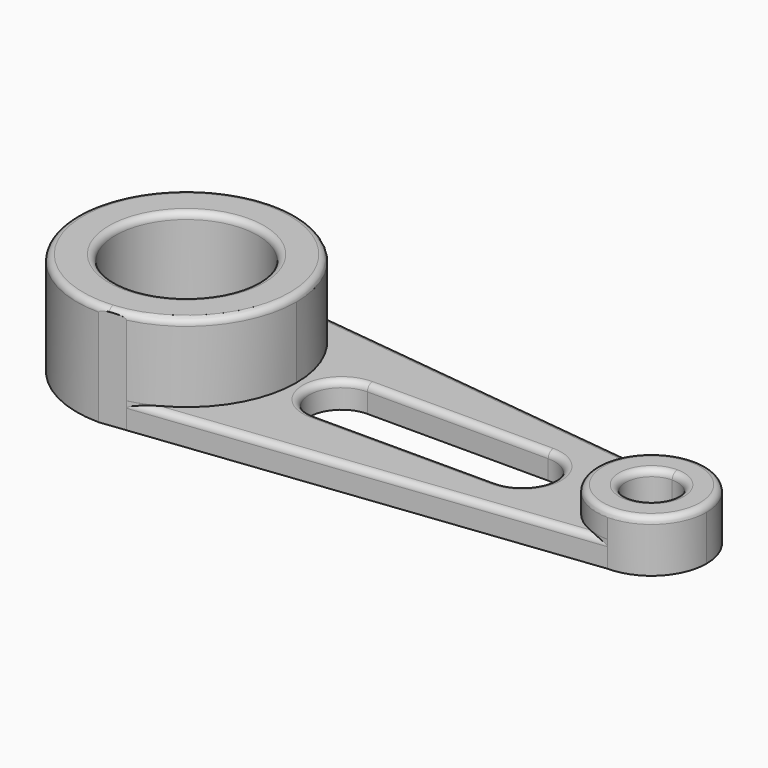
from build123d import *

# Parameters (mm, degrees)
F0_R         = 34.925
F1_DEPTH     = 50.8
F2_DEPTH     = 12.7
F3_DEPTH     = 25.4
F4_T2_ANGLE  = 170.0024112312
F4_T4_ANGLE  = 196.8788005765
F4_T8_DEPTH  = 281.0532283158
F4_S9_R      = 27.051
F4_T10_DEPTH = 142
F4_S11_R     = 53.975
F4_T12_DEPTH = 142
F4_T16_DEPTH = 281.0532283158
F4_S17_R     = 27.051
F4_T18_DEPTH = 142
F4_S19_R     = 53.975
F4_T20_DEPTH = 142
F5_R         = 3.175


# Not quite as in the source:
# - a fillet or chamfer that OpenCascade refuses, or shapes differently, is made with other operations: its cross-section is extruded or revolved along the edge and cut away or added


with BuildPart() as f1:
    # F0 (on Top) → F1 (new body)
    with BuildSketch(Plane.XY):
        with BuildLine():
            Line((-131.9052666893, 52.4980479424), (-144.4454256691, 53.975))
            ThreePointArc((-144.4454256691, 53.975), (-198.4204256691, 0), (-144.4454256691, -53.975))
            Line((-144.4454256691, -53.975), (-131.9052666893, -52.4980479424))
            ThreePointArc((-131.9052666893, -52.4980479424), (-102.0770665674, -33.4398380981), (-90.4704256691, 0))
            ThreePointArc((-90.4704256691, 0), (-102.0770665674, 33.4398380981), (-131.9052666893, 52.4980479424))
        make_face()
        with Locations((-144.4454256691, 0)):
            Circle(F0_R, mode=Mode.SUBTRACT)
    extrude(amount=F1_DEPTH)

    # F0 (on Top) → F2 (join)
    with BuildSketch(Plane.XY):
        with BuildLine():
            Line((84.1545743309, 27.051), (-131.9052666893, 52.4980479424))
            ThreePointArc((-131.9052666893, 52.4980479424), (-102.0770665674, 33.4398380981), (-90.4704256691, 0))
            ThreePointArc((-90.4704256691, 0), (-102.0770665674, -33.4398380981), (-131.9052666893, -52.4980479424))
            Line((-131.9052666893, -52.4980479424), (84.1545743309, -27.051))
            ThreePointArc((84.1545743309, -27.051), (57.1035743309, 0), (84.1545743309, 27.051))
        make_face()
        with BuildLine():
            ThreePointArc((-68.2454256691, -15.875), (-84.1204256691, 0), (-68.2454256691, 15.875))
            Line((-68.2454256691, 15.875), (20.6545743309, 15.875))
            ThreePointArc((20.6545743309, 15.875), (36.5295743309, 0), (20.6545743309, -15.875))
            Line((20.6545743309, -15.875), (-68.2454256691, -15.875))
        make_face(mode=Mode.SUBTRACT)
    extrude(amount=F2_DEPTH)

    # F0 (on Top) → F3 (join)
    with BuildSketch(Plane.XY):
        with BuildLine():
            ThreePointArc((111.2055743309, 0), (103.2825198687, 19.1279455379), (84.1545743309, 27.051))
            Line((84.1545743309, 27.051), (84.1545743309, 12.7))
            ThreePointArc((84.1545743309, 12.7), (93.1348304519, 8.9802561211), (96.8545743309, 0))
            ThreePointArc((96.8545743309, 0), (93.1348304519, -8.9802561211), (84.1545743309, -12.7))
            Line((84.1545743309, -12.7), (84.1545743309, -27.051))
            ThreePointArc((84.1545743309, -27.051), (103.2825198687, -19.1279455379), (111.2055743309, 0))
        make_face()
        with BuildLine():
            Line((84.1545743309, 12.7), (84.1545743309, 27.051))
            ThreePointArc((84.1545743309, 27.051), (57.1035743309, 0), (84.1545743309, -27.051))
            Line((84.1545743309, -27.051), (84.1545743309, -12.7))
            ThreePointArc((84.1545743309, -12.7), (71.4545743309, 0), (84.1545743309, 12.7))
        make_face()
    extrude(amount=F3_DEPTH)

    # F4: fillet of radius 3.175 on 5 edges, made by hand

    # F4_s1 → F4_t2 (revolve, cut)
    with BuildSketch(Plane(origin=(-143.3487281035, 12.5383492192, 0), x_dir=(0, 0, 1), z_dir=(-0.9961965318, 0.0871347808, 0))):
        with BuildLine():
            ThreePointArc((47.625, 41.3887794913), (49.8700640303, 40.4588435216), (50.8, 38.2137794913))
            Line((50.8, 38.2137794913), (50.8635, 38.2137794913))
            Line((50.8635, 38.2137794913), (50.8635, 41.4522794913))
            Line((50.8635, 41.4522794913), (47.625, 41.4522794913))
            Line((47.625, 41.4522794913), (47.625, 41.3887794913))
        make_face()
    revolve(axis=Axis((-144.4454256691, 0, 50.8), (0, 0, -1)), revolution_arc=F4_T2_ANGLE, mode=Mode.SUBTRACT)

    # F4_s3 → F4_t4 (revolve, cut)
    with BuildSketch(Plane(origin=(-141.3341490778, 20.9697312712, 0), x_dir=(0, 0, 1), z_dir=(0.9891716429, -0.1467632817, 0))):
        with BuildLine():
            ThreePointArc((50.8, -29.6007153042), (49.8700640303, -31.8457793344), (47.625, -32.7757153042))
            Line((47.625, -32.7757153042), (47.625, -32.8392153042))
            Line((47.625, -32.8392153042), (50.8635, -32.8392153042))
            Line((50.8635, -32.8392153042), (50.8635, -29.6007153042))
            Line((50.8635, -29.6007153042), (50.8, -29.6007153042))
        make_face()
    revolve(axis=Axis((-144.4454256691, 0, 50.8), (0, 0, 1)), revolution_arc=F4_T4_ANGLE, mode=Mode.SUBTRACT)


with BuildPart() as f4_tool6:
    # F4_s7 → F4_t8 (new body)
    with BuildSketch(Plane(origin=(-175.6141368199, -20.683442781, 0), x_dir=(0, 0, 1), z_dir=(0.9931355314, 0.1169692959, 0))):
        with BuildLine():
            ThreePointArc((12.7, 33.5338105694), (11.7700640303, 35.7788745997), (9.525, 36.7088105694))
            Line((9.525, 36.7088105694), (9.525, 36.7723105694))
            Line((9.525, 36.7723105694), (12.7635, 36.7723105694))
            Line((12.7635, 36.7723105694), (12.7635, 33.5338105694))
            Line((12.7635, 33.5338105694), (12.7, 33.5338105694))
        make_face()
    extrude(amount=F4_T8_DEPTH)

    # F4_s9 → F4_t10 (cut, symmetric)
    with BuildSketch(Plane.XY.offset(11.1)):
        with Locations((84.1545743309, 0)):
            Circle(F4_S9_R)
    extrude(amount=F4_T10_DEPTH, both=True, mode=Mode.SUBTRACT)

    # F4_s11 → F4_t12 (cut, symmetric)
    with BuildSketch(Plane.XY.offset(11.1)):
        with Locations((-144.4454256691, 0)):
            Circle(F4_S11_R)
    extrude(amount=F4_T12_DEPTH, both=True, mode=Mode.SUBTRACT)


with BuildPart() as f1_1:
    add(f1.part)

    # F4_t5: cut F4_tool6
    add(f4_tool6.part, mode=Mode.SUBTRACT)


with BuildPart() as f4_tool14:
    # F4_s15 → F4_t16 (new body)
    with BuildSketch(Plane(origin=(103.5098104467, -12.1911554526, 0), x_dir=(0, 0, 1), z_dir=(-0.9931355314, 0.1169692959, 0))):
        with BuildLine():
            ThreePointArc((9.525, 36.7088105694), (11.7700640303, 35.7788745997), (12.7, 33.5338105694))
            Line((12.7, 33.5338105694), (12.7635, 33.5338105694))
            Line((12.7635, 33.5338105694), (12.7635, 36.7723105694))
            Line((12.7635, 36.7723105694), (9.525, 36.7723105694))
            Line((9.525, 36.7723105694), (9.525, 36.7088105694))
        make_face()
    extrude(amount=F4_T16_DEPTH)

    # F4_s17 → F4_t18 (cut, symmetric)
    with BuildSketch(Plane.XY.offset(11.1)):
        with Locations((84.1545743309, 0)):
            Circle(F4_S17_R)
    extrude(amount=F4_T18_DEPTH, both=True, mode=Mode.SUBTRACT)

    # F4_s19 → F4_t20 (cut, symmetric)
    with BuildSketch(Plane.XY.offset(11.1)):
        with Locations((-144.4454256691, 0)):
            Circle(F4_S19_R)
    extrude(amount=F4_T20_DEPTH, both=True, mode=Mode.SUBTRACT)


with BuildPart() as f1_2:
    add(f1_1.part)

    # F4_t13: cut F4_tool14
    add(f4_tool14.part, mode=Mode.SUBTRACT)

    # F4_s21 → F4_t22 (revolve, cut)
    with BuildSketch(Plane.XZ):
        with BuildLine():
            ThreePointArc((111.2055743309, 22.225), (110.2756383611, 24.4700640303), (108.0305743309, 25.4))
            Line((108.0305743309, 25.4), (108.0305743309, 25.4635))
            Line((108.0305743309, 25.4635), (111.2690743309, 25.4635))
            Line((111.2690743309, 25.4635), (111.2690743309, 22.225))
            Line((111.2690743309, 22.225), (111.2055743309, 22.225))
        make_face()
    revolve(axis=Axis((84.1545743309, 0, 25.4), (0, 0, 1)), mode=Mode.SUBTRACT)

    # F5
    f5_edges = [f1_2.edges().sort_by_distance(p)[0] for p in [
        (-179.370426, 0, 50.8),
        (-23.795426, -15.875, 12.7),
        (96.854574, 0, 12.7),
        (71.454574, 0, 0),
        (71.454574, 0, 25.4),
        (36.529574, 0, 12.7),
        (-23.795426, 15.875, 12.7),
        (-84.120426, 0, 12.7),
    ]]
    fillet(f5_edges, radius=F5_R)


solid = f1_2.part
